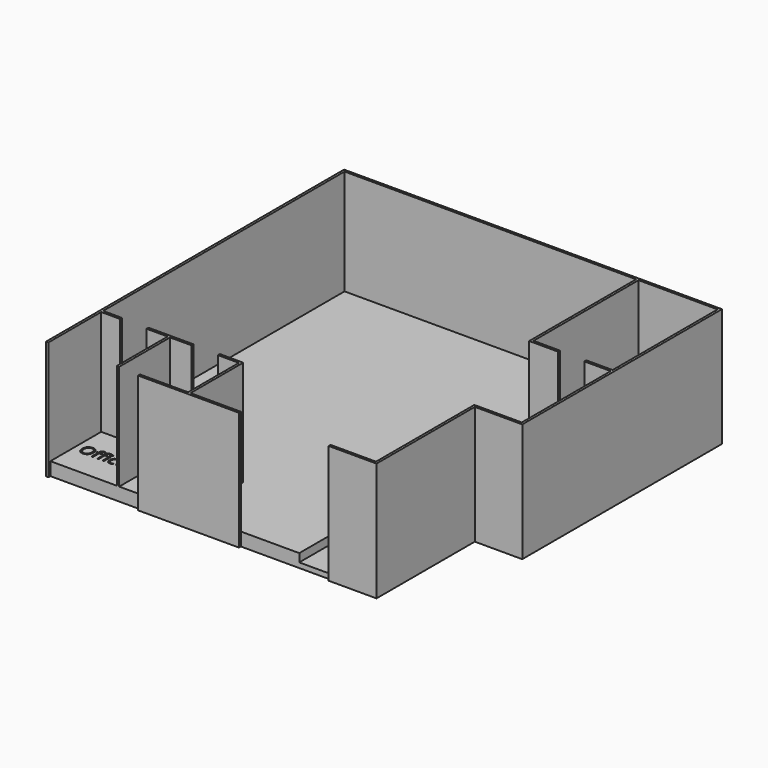
from build123d import *

# Parameters (mm, degrees)
F0_W            = 14330
F0_H            = 14125
F1_DEPTH        = 500
F2_W            = 14150
F2_H            = 13945
F3_DEPTH        = 4000
F4_W            = 3400
F4_H            = 90
F5_DEPTH        = 4820
F6_W            = 3000
F6_H            = 4570
F7_DEPTH        = 310
F8_W            = 1896.4712715149
F8_H            = 4783.384475708
F9_DEPTH        = 1900
F9_DEPTH_BACK   = 5000
F11_DEPTH       = 4000
F11_DEPTH_BACK  = 440
F13_DEPTH       = 4000
F15_DEPTH       = 4000
F16_W           = 1000
F16_H           = 90
F17_DEPTH       = 4000
F18_TEXT_SIZE   = 495.8154272823
F18_TEXT_SIZE_2 = 637.4201993982
F18_TEXT_SIZE_3 = 673.8412864512
F19_DEPTH       = 120
F20_TEXT_SIZE   = 966.2827677882
F21_DEPTH       = 25


# Not quite as in the source:
# - Text() gives the source's letters only with a copy of the font that has no kerning and outlines rounded to 1/6400 em; it was checked with that copy


with BuildPart() as f1:
    # F0 (on Top) → F1 (new body)
    with BuildSketch(Plane.XY):
        Rectangle(F0_W, F0_H)
    extrude(amount=F1_DEPTH)

    # F2 (on face) → F3 (join)
    with BuildSketch(Plane.XY.offset(500)):
        Polygon((7165, 7062.5), (-7165, 7062.5), (-7165, 6972.5), (-7165, 6847.5), (-7165, -6972.5), (-7165, -7062.5), (7075, -7062.5), (7165, -7062.5), (7165, 6972.5), align=None)
        Rectangle(F2_W, F2_H, mode=Mode.SUBTRACT)
    extrude(amount=F3_DEPTH)

    # F4 (on face) → F5 (cut)
    with BuildSketch(Plane.XY.offset(4500)):
        with Locations((-5375, -7017.5)):
            Rectangle(F4_W, F4_H)
        with Locations((1850, -7017.5)):
            Rectangle(F4_W, F4_H)
    extrude(amount=-F5_DEPTH, mode=Mode.SUBTRACT)

    # F6 (on face) → F7 (cut)
    with BuildSketch(Plane.XY.offset(500)):
        with Locations((3865, -4687.5)):
            Rectangle(F6_W, F6_H)
    extrude(amount=-F7_DEPTH, mode=Mode.SUBTRACT)

    # F8 (on face) → F9 (cut, two sides)
    with BuildSketch(Plane.XY.offset(500)) as f9_sk:
        with Locations((6313.2356357574, -4794.192237854)):
            Rectangle(F8_W, F8_H)
    extrude(amount=-F9_DEPTH, mode=Mode.SUBTRACT)
    extrude(f9_sk.sketch, amount=F9_DEPTH_BACK, mode=Mode.SUBTRACT)

    # F10 (on face) → F11 (join, two sides)
    with BuildSketch(Plane.XY.offset(500)) as f11_sk:
        Polygon((5365, -2402.5), (7075, -2402.5), (7075, -2312.5), (5365, -2312.5), (5275, -2312.5), (5275, -7036.1723899841), (5365, -7036.1723899841), align=None)
    extrude(amount=F11_DEPTH)
    extrude(f11_sk.sketch, amount=-F11_DEPTH_BACK)

    # F12 (on face) → F13 (join)
    with BuildSketch(Plane.XY.offset(500)):
        Polygon((7075, 1902.7505146229), (7075, 1992.7505146229), (4075, 1992.7505146229), (4075, 6992.7505146229), (3985, 6972.5), (3985, 1902.7505146229), align=None)
    extrude(amount=F13_DEPTH)

    # F14 (on face) → F15 (join)
    with BuildSketch(Plane.XY.offset(500)):
        Polygon((-7075, -4472.5), (-7075, -4562.5), (-4553.75, -4562.5), (-4553.75, -6972.5), (-4463.75, -6972.5), (-4463.75, -4562.5), (-1852.5, -4562.5), (-1852.5, -6972.5), (-1762.5, -6972.5), (-1762.5, -4472.5), align=None)
    extrude(amount=F15_DEPTH)

    # F16 (on face) → F17 (cut)
    with BuildSketch(Plane.XY.offset(4500)):
        with Locations((-5853.75, -4517.5)):
            Rectangle(F16_W, F16_H)
        with Locations((-3152.5, -4517.5)):
            Rectangle(F16_W, F16_H)
        with Locations((5575, 1947.7505146229)):
            Rectangle(F16_W, F16_H)
    extrude(amount=-F17_DEPTH, mode=Mode.SUBTRACT)

    # F18 (on face) → F19 (cut)
    with BuildSketch(Plane.XY.offset(500)):
        with Locations((4275, 4736.6371702011)):
            Text('Conference', F18_TEXT_SIZE, font='Open Sans', text_align=(TextAlign.LEFT, TextAlign.BOTTOM))
        with Locations((4275, 4062.3281890971)):
            Text('Room', F18_TEXT_SIZE, font='Open Sans', text_align=(TextAlign.LEFT, TextAlign.BOTTOM))
        with Locations((-6875, -5982.1925163269)):
            Text('Office 1', F18_TEXT_SIZE_2, font='Open Sans', text_align=(TextAlign.LEFT, TextAlign.BOTTOM))
        with Locations((-4263.75, -6008.4156990051)):
            Text('Office 2', F18_TEXT_SIZE_3, font='Open Sans', text_align=(TextAlign.LEFT, TextAlign.BOTTOM))
    extrude(amount=-F19_DEPTH, mode=Mode.SUBTRACT)

    # F20 (on face) → F21 (cut)
    with BuildSketch(Plane.XY.offset(190)):
        with Locations((2565, -5147.2603332092)):
            Text('Stairs', F20_TEXT_SIZE, font='Open Sans', text_align=(TextAlign.LEFT, TextAlign.BOTTOM))
    extrude(amount=-F21_DEPTH, mode=Mode.SUBTRACT)


solid = f1.part
